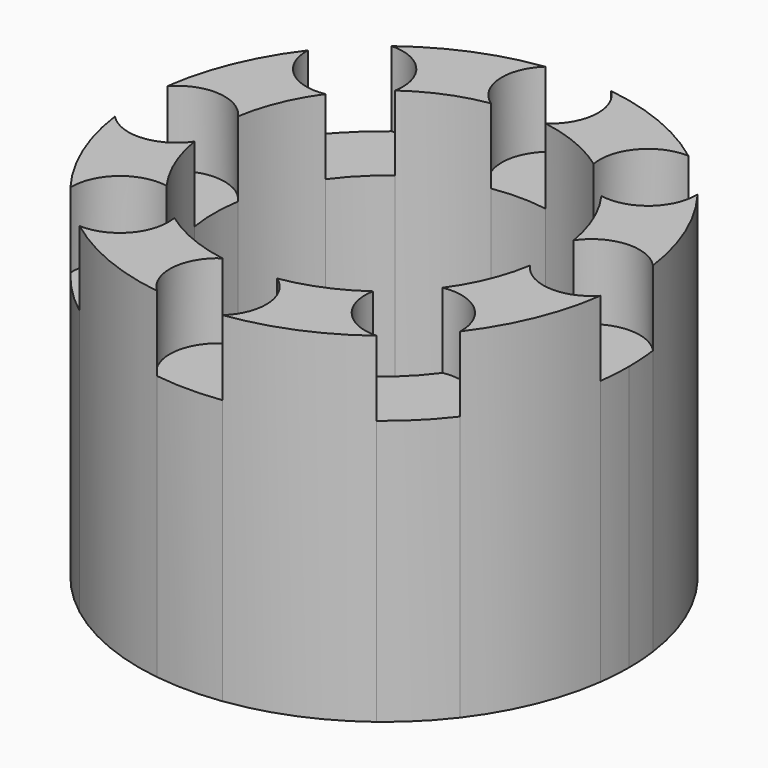
from build123d import *

# Parameters (mm, degrees)
F1_DEPTH = 3.175
F2_DEPTH = 2.475


# Not quite as in the source:
# - a length typed as a fraction of an inch, garbled in the dataset ("3 / 203.2 mm" for 3/8 in), is restored


with BuildPart() as f1:
    # F0 (on Top) → F1 (new body)
    with BuildSketch(Plane.XY):
        with BuildLine():
            ThreePointArc((-1.5668548387, -6.0323095527), (-1.4666587579, -5.6799900511), (-1.2883805774, -5.3600132142))
            ThreePointArc((-1.2883805774, -5.3600132142), (-1.6640391224, -5.2581452502), (-1.8197325394, -4.9014156826))
            ThreePointArc((-1.8197325394, -4.9014156826), (-2.1133744306, -5.4121116485), (-2.2668548387, -5.9808644016))
            ThreePointArc((-2.2668548387, -5.9808644016), (-1.9045170714, -5.8387103762), (-1.5668548387, -6.0323095527))
        make_face()
    extrude(amount=F1_DEPTH)



with BuildPart() as f1b:
    # F0 (on Top) → F1, piece 2 (new body)
    with BuildSketch(Plane.XY):
        with BuildLine():
            ThreePointArc((-0.9274867858, -4.9991194226), (-0.6075099489, -4.8208412421), (-0.2551904473, -4.7206451613))
            ThreePointArc((-0.2551904473, -4.7206451613), (-0.4487896238, -4.3829829286), (-0.3066355984, -4.0206451613))
            ThreePointArc((-0.3066355984, -4.0206451613), (-0.8753883515, -4.1741255694), (-1.3860843174, -4.4677674606))
            ThreePointArc((-1.3860843174, -4.4677674606), (-1.0575527647, -4.5936525568), (-0.9200193885, -4.9174806115))
            ThreePointArc((-0.9200193885, -4.9174806115), (-0.9218901264, -4.9584704197), (-0.9274867858, -4.9991194226))
        make_face()
    extrude(amount=F1_DEPTH)


with BuildPart() as f1c:
    # F0 (on Top) → F1, piece 3 (new body)
    with BuildSketch(Plane.XY):
        with BuildLine():
            ThreePointArc((0.2551904473, -4.7206451613), (0.6075099489, -4.8208412421), (0.9274867858, -4.9991194226))
            ThreePointArc((0.9274867858, -4.9991194226), (1.0293547498, -4.6234608776), (1.3860843174, -4.4677674606))
            ThreePointArc((1.3860843174, -4.4677674606), (0.8753883515, -4.1741255694), (0.3066355984, -4.0206451613))
            ThreePointArc((0.3066355984, -4.0206451613), (0.4126051498, -4.1703976883), (0.45, -4.35))
            ThreePointArc((0.45, -4.35), (0.3983313328, -4.559361289), (0.2551904473, -4.7206451613))
        make_face()
    extrude(amount=F1_DEPTH)


with BuildPart() as f1d:
    # F0 (on Top) → F1, piece 4 (new body)
    with BuildSketch(Plane.XY):
        with BuildLine():
            ThreePointArc((1.2883805774, -5.3600132142), (1.4666587579, -5.6799900511), (1.5668548387, -6.0323095527))
            ThreePointArc((1.5668548387, -6.0323095527), (1.9045170714, -5.8387103762), (2.2668548387, -5.9808644016))
            ThreePointArc((2.2668548387, -5.9808644016), (2.1133744306, -5.4121116485), (1.8197325394, -4.9014156826))
            ThreePointArc((1.8197325394, -4.9014156826), (1.8199476706, -4.9094468667), (1.8200193885, -4.9174806115))
            ThreePointArc((1.8200193885, -4.9174806115), (1.6579104573, -5.2633400229), (1.2883805774, -5.3600132142))
        make_face()
    extrude(amount=F1_DEPTH)


with BuildPart() as f1e:
    # F0 (on Top) → F1, piece 5 (new body)
    with BuildSketch(Plane.XY):
        with BuildLine():
            ThreePointArc((2.2668548387, -6.5941355984), (1.9045170714, -6.7362896238), (1.5668548387, -6.5426904473))
            ThreePointArc((1.5668548387, -6.5426904473), (1.4666587579, -6.8950099489), (1.2883805774, -7.2149867858))
            ThreePointArc((1.2883805774, -7.2149867858), (1.6579104573, -7.3116599771), (1.8200193885, -7.6575193885))
            ThreePointArc((1.8200193885, -7.6575193885), (1.8199476706, -7.6655531333), (1.8197325394, -7.6735843174))
            ThreePointArc((1.8197325394, -7.6735843174), (2.1133744306, -7.1628883515), (2.2668548387, -6.5941355984))
        make_face()
    extrude(amount=F1_DEPTH)


with BuildPart() as f1f:
    # F0 (on Top) → F1, piece 6 (new body)
    with BuildSketch(Plane.XY):
        with BuildLine():
            ThreePointArc((1.3860843174, -8.1072325394), (1.0293547498, -7.9515391224), (0.9274867858, -7.5758805774))
            ThreePointArc((0.9274867858, -7.5758805774), (0.6075099489, -7.7541587579), (0.2551904473, -7.8543548387))
            ThreePointArc((0.2551904473, -7.8543548387), (0.3983313328, -8.015638711), (0.45, -8.225))
            ThreePointArc((0.45, -8.225), (0.4126051498, -8.4046023117), (0.3066355984, -8.5543548387))
            ThreePointArc((0.3066355984, -8.5543548387), (0.8753883515, -8.4008744306), (1.3860843174, -8.1072325394))
        make_face()
    extrude(amount=F1_DEPTH)


with BuildPart() as f1g:
    # F0 (on Top) → F1, piece 7 (new body)
    with BuildSketch(Plane.XY):
        with BuildLine():
            ThreePointArc((-0.3066355984, -8.5543548387), (-0.4487896238, -8.1920170714), (-0.2551904473, -7.8543548387))
            ThreePointArc((-0.2551904473, -7.8543548387), (-0.6075099489, -7.7541587579), (-0.9274867858, -7.5758805774))
            ThreePointArc((-0.9274867858, -7.5758805774), (-0.9218901264, -7.6165295803), (-0.9200193885, -7.6575193885))
            ThreePointArc((-0.9200193885, -7.6575193885), (-1.0575527647, -7.9813474432), (-1.3860843174, -8.1072325394))
            ThreePointArc((-1.3860843174, -8.1072325394), (-0.8753883515, -8.4008744306), (-0.3066355984, -8.5543548387))
        make_face()
    extrude(amount=F1_DEPTH)


with BuildPart() as f1h:
    # F0 (on Top) → F1, piece 8 (new body)
    with BuildSketch(Plane.XY):
        with BuildLine():
            ThreePointArc((-1.8197325394, -7.6735843174), (-1.6640391224, -7.3168547498), (-1.2883805774, -7.2149867858))
            ThreePointArc((-1.2883805774, -7.2149867858), (-1.4666587579, -6.8950099489), (-1.5668548387, -6.5426904473))
            ThreePointArc((-1.5668548387, -6.5426904473), (-1.9045170714, -6.7362896238), (-2.2668548387, -6.5941355984))
            ThreePointArc((-2.2668548387, -6.5941355984), (-2.1133744306, -7.1628883515), (-1.8197325394, -7.6735843174))
        make_face()
    extrude(amount=F1_DEPTH)


with BuildPart() as f1_1:
    add(f1.part)

    add(f1b.part)  # F2 merges F1b

    add(f1c.part)  # F2 merges F1c

    add(f1d.part)  # F2 merges F1d

    add(f1e.part)  # F2 merges F1e

    add(f1f.part)  # F2 merges F1f

    add(f1g.part)  # F2 merges F1g

    add(f1h.part)  # F2 merges F1h
    # F0 (on Top) → F2 (join)
    with BuildSketch(Plane.XY):
        with BuildLine():
            ThreePointArc((-1.2883805774, -5.3600132142), (-1.1225320151, -5.1649679849), (-0.9274867858, -4.9991194226))
            ThreePointArc((-0.9274867858, -4.9991194226), (-0.9218901264, -4.9584704197), (-0.9200193885, -4.9174806115))
            ThreePointArc((-0.9200193885, -4.9174806115), (-1.0575527647, -4.5936525568), (-1.3860843174, -4.4677674606))
            ThreePointArc((-1.3860843174, -4.4677674606), (-1.617506762, -4.669993238), (-1.8197325394, -4.9014156826))
            ThreePointArc((-1.8197325394, -4.9014156826), (-1.6640391224, -5.2581452502), (-1.2883805774, -5.3600132142))
        make_face()
        with BuildLine():
            ThreePointArc((-0.2551904473, -4.7206451613), (0, -4.7), (0.2551904473, -4.7206451613))
            ThreePointArc((0.2551904473, -4.7206451613), (0.3983313328, -4.559361289), (0.45, -4.35))
            ThreePointArc((0.45, -4.35), (0.4126051498, -4.1703976883), (0.3066355984, -4.0206451613))
            ThreePointArc((0.3066355984, -4.0206451613), (0, -4), (-0.3066355984, -4.0206451613))
            ThreePointArc((-0.3066355984, -4.0206451613), (-0.4487896238, -4.3829829286), (-0.2551904473, -4.7206451613))
        make_face()
        with BuildLine():
            ThreePointArc((0.9274867858, -4.9991194226), (1.1225320151, -5.1649679849), (1.2883805774, -5.3600132142))
            ThreePointArc((1.2883805774, -5.3600132142), (1.6579104573, -5.2633400229), (1.8200193885, -4.9174806115))
            ThreePointArc((1.8200193885, -4.9174806115), (1.8199476706, -4.9094468667), (1.8197325394, -4.9014156826))
            ThreePointArc((1.8197325394, -4.9014156826), (1.617506762, -4.669993238), (1.3860843174, -4.4677674606))
            ThreePointArc((1.3860843174, -4.4677674606), (1.0293547498, -4.6234608776), (0.9274867858, -4.9991194226))
        make_face()
        with BuildLine():
            ThreePointArc((1.5668548387, -6.0323095527), (1.5823302921, -6.1594879038), (1.5875, -6.2875))
            ThreePointArc((1.5875, -6.2875), (1.5823302921, -6.4155120962), (1.5668548387, -6.5426904473))
            ThreePointArc((1.5668548387, -6.5426904473), (1.9045170714, -6.7362896238), (2.2668548387, -6.5941355984))
            ThreePointArc((2.2668548387, -6.5941355984), (2.2823328738, -6.4411649056), (2.2875, -6.2875))
            ThreePointArc((2.2875, -6.2875), (2.2823328738, -6.1338350944), (2.2668548387, -5.9808644016))
            ThreePointArc((2.2668548387, -5.9808644016), (1.9045170714, -5.8387103762), (1.5668548387, -6.0323095527))
        make_face()
        with BuildLine():
            ThreePointArc((1.8200193885, -7.6575193885), (1.6579104573, -7.3116599771), (1.2883805774, -7.2149867858))
            ThreePointArc((1.2883805774, -7.2149867858), (1.1225320151, -7.4100320151), (0.9274867858, -7.5758805774))
            ThreePointArc((0.9274867858, -7.5758805774), (1.0293547498, -7.9515391224), (1.3860843174, -8.1072325394))
            ThreePointArc((1.3860843174, -8.1072325394), (1.617506762, -7.905006762), (1.8197325394, -7.6735843174))
            ThreePointArc((1.8197325394, -7.6735843174), (1.8199476706, -7.6655531333), (1.8200193885, -7.6575193885))
        make_face()
        with BuildLine():
            ThreePointArc((0.45, -8.225), (0.3983313328, -8.015638711), (0.2551904473, -7.8543548387))
            ThreePointArc((0.2551904473, -7.8543548387), (0, -7.875), (-0.2551904473, -7.8543548387))
            ThreePointArc((-0.2551904473, -7.8543548387), (-0.4487896238, -8.1920170714), (-0.3066355984, -8.5543548387))
            ThreePointArc((-0.3066355984, -8.5543548387), (0, -8.575), (0.3066355984, -8.5543548387))
            ThreePointArc((0.3066355984, -8.5543548387), (0.4126051498, -8.4046023117), (0.45, -8.225))
        make_face()
        with BuildLine():
            ThreePointArc((-0.9200193885, -7.6575193885), (-0.9218901264, -7.6165295803), (-0.9274867858, -7.5758805774))
            ThreePointArc((-0.9274867858, -7.5758805774), (-1.1225320151, -7.4100320151), (-1.2883805774, -7.2149867858))
            ThreePointArc((-1.2883805774, -7.2149867858), (-1.6640391224, -7.3168547498), (-1.8197325394, -7.6735843174))
            ThreePointArc((-1.8197325394, -7.6735843174), (-1.617506762, -7.905006762), (-1.3860843174, -8.1072325394))
            ThreePointArc((-1.3860843174, -8.1072325394), (-1.0575527647, -7.9813474432), (-0.9200193885, -7.6575193885))
        make_face()
        with BuildLine():
            ThreePointArc((-1.5668548387, -6.5426904473), (-1.5875, -6.2875), (-1.5668548387, -6.0323095527))
            ThreePointArc((-1.5668548387, -6.0323095527), (-1.9045170714, -5.8387103762), (-2.2668548387, -5.9808644016))
            ThreePointArc((-2.2668548387, -5.9808644016), (-2.2875, -6.2875), (-2.2668548387, -6.5941355984))
            ThreePointArc((-2.2668548387, -6.5941355984), (-1.9045170714, -6.7362896238), (-1.5668548387, -6.5426904473))
        make_face()
    extrude(amount=F2_DEPTH)


solid = f1_1.part
